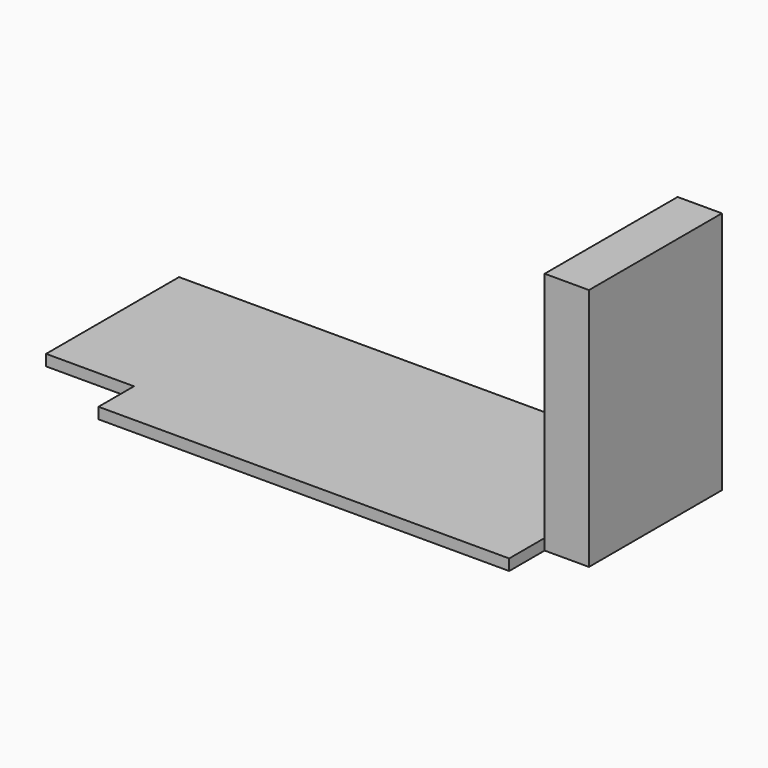
from build123d import *

# Parameters (mm, degrees)
F1_DEPTH = 22
F2_DEPTH = 1


with BuildPart() as f1:
    # F0 (on Top) → F1 (new body)
    with BuildSketch(Plane.XY):
        Polygon((41.0671858334, 12.6168608051), (37.0671858334, 12.6168608051), (37.0671858334, 8.6168608051), (37.0671858334, -2.3831391949), (41.0671858334, -2.3831391949), align=None)
    extrude(amount=F1_DEPTH)


with BuildPart() as f2:
    # F0 (on Top) → F2 (new body)
    with BuildSketch(Plane.XY):
        Polygon((37.0671858334, 12.6168608051), (-7.9328141666, 12.6168608051), (-7.9328141666, -2.3831391949), (0, -2.3831391949), (0, -6.3831391949), (37.0671858334, -6.3831391949), (37.0671858334, -2.3831391949), (37.0671858334, 8.6168608051), align=None)
    extrude(amount=F2_DEPTH)


solid = Compound([f1.part, f2.part])
